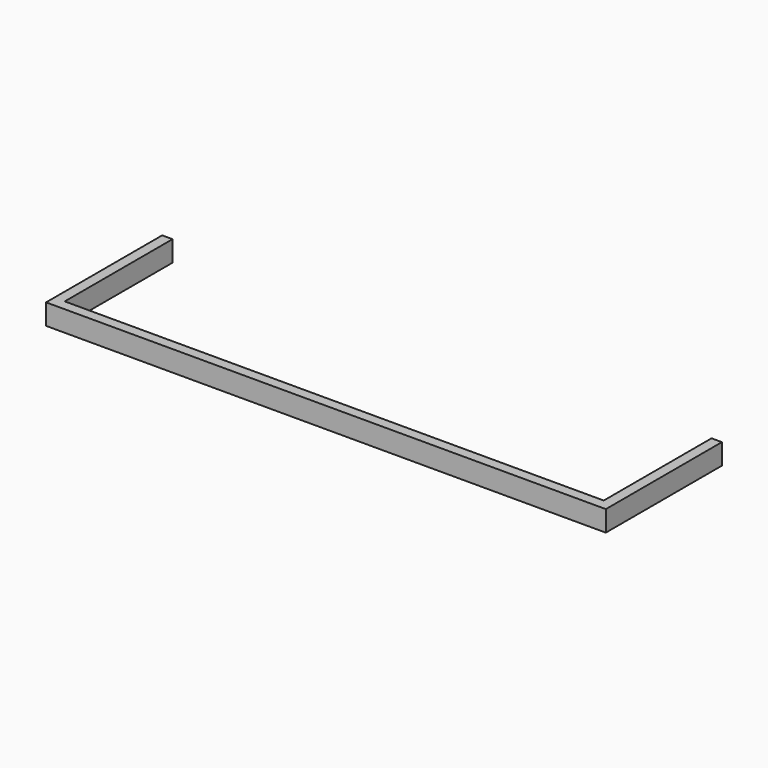
from build123d import *

# Parameters (mm, degrees)
F0_W          = 108
F0_H          = 30
F1_DEPTH      = 2
F3_DEPTH      = 39
F5_DEPTH      = 30.001
F6_DEPTH      = 4
F7_ANGLE      = -90
F8_T1_DEPTH   = 104
F8_T3_DEPTH   = 39
F8_T9_DEPTH   = 116.5
F8_T13_DEPTH  = 51.5
F8_T20_DEPTH  = 116.5
F8_T24_DEPTH  = 51.5
F9_R          = 2.55
F10_DEPTH     = 2.0010001
F15_TEXT_SIZE = 6.25
F16_DEPTH     = 0.7
F18_DEPTH     = 2


# Not quite as in the source:
# - a fillet or chamfer that OpenCascade refuses, or shapes differently, is made with other operations: its cross-section is extruded or revolved along the edge and cut away or added
# - a feature of the source that left no trace in its solid (it failed there, or was rolled back) is left out
# - Text() gives the source's letters only with a copy of the font that has no kerning and outlines rounded to 1/6400 em; it was checked with that copy


with BuildPart() as f1:
    # F0 (on Top) → F1 (new body)
    with BuildSketch(Plane.XY):
        with Locations((54, -15)):
            Rectangle(F0_W, F0_H)
    extrude(amount=-F1_DEPTH)

    # F2 (on face) → F3 (join)
    with BuildSketch(Plane(origin=(0, 0, -2), x_dir=(1, 0, 0), z_dir=(0, 0, -1))):
        Polygon((2, 28), (106, 28), (106, 2), (108, 2), (108, 30), (0, 30), (0, 2), (2, 2), align=None)
    extrude(amount=F3_DEPTH)

    # F4 (on face) → F5 (cut, through all)
    with BuildSketch(Plane.XZ.offset(30)):
        with BuildLine():
            Line((21.7352903846, -5.3176150288), (31.189246754, -24.36107081))
            ThreePointArc((31.189246754, -24.36107081), (22.5427599741, -36.7534160144), (37.0153844173, -32.408868279))
            Line((37.0153844173, -32.408868279), (35.7390828431, -20.9399661981))
            add(Edge.make_bspline(
                [(35.7390828431, -20.9399661981), (40.0774041837, -22.3301620555), (41.4828972701, -14.9319285827), (53.2948829776, -15.8111795219), (53.9903119206, -20.9399661981)],
                knots=[0, 0, 0, 0, 0.4737528897, 1, 1, 1, 1], degree=3))
            add(Edge.make_bspline(
                [(35.3899858892, -8.0947782844), (38.894245401, -7.2189187631), (48.5971156185, -8.2695706), (55.5558682276, -17.4074323859), (53.9903119206, -20.9399661981)],
                knots=[0, 0, 0, 0, 0.5069746376, 1, 1, 1, 1], degree=3))
            add(Edge.make_bspline(
                [(21.7352903846, -5.3176150288), (23.8003305692, -7.4651161077), (28.3369070804, -10.5817247057), (34.3228683985, -8.1395113196), (35.3899858892, -8.0947782844)],
                knots=[0, 0, 0, 0, 0.5306283003, 1, 1, 1, 1], degree=3))
        make_face()
    extrude(amount=-F5_DEPTH, mode=Mode.SUBTRACT)


with BuildPart() as f6:
    # F6 (new): a face of the model
    f6_faces = [f1.part.faces().sort_by_distance(p)[0] for p in [
        (54, -29.1157060545, -41),
    ]]
    extrude(f6_faces, amount=F6_DEPTH)


with BuildPart() as f1_1:
    # F7: moved
    add(f1.part.rotate(Axis((54, -30, -41), (-1, 0, 0)), F7_ANGLE))

    # F8: fillet of radius 5 on 3 edges, made by hand

    # F8_s2 → F8_t1 (join)
    with BuildSketch(Plane.YZ.offset(2)):
        with BuildLine():
            ThreePointArc((-69, -34), (-67.5355339059, -37.5355339059), (-64, -39))
            Line((-64, -39), (-64, -39.1))
            Line((-64, -39.1), (-69.1, -39.1))
            Line((-69.1, -39.1), (-69.1, -34))
            Line((-69.1, -34), (-69, -34))
        make_face()
    extrude(amount=F8_T1_DEPTH)

    # F8_s4 → F8_t3 (join)
    with BuildSketch(Plane.XZ.offset(30)):
        with BuildLine():
            ThreePointArc((7, -39), (3.4644660941, -37.5355339059), (2, -34))
            Line((2, -34), (1.9, -34))
            Line((1.9, -34), (1.9, -39.1))
            Line((1.9, -39.1), (7, -39.1))
            Line((7, -39.1), (7, -39))
        make_face()
        with BuildLine():
            ThreePointArc((101, -39), (104.5355339059, -37.5355339059), (106, -34))
            Line((106, -34), (106.1, -34))
            Line((106.1, -34), (106.1, -39.1))
            Line((106.1, -39.1), (101, -39.1))
            Line((101, -39.1), (101, -39))
        make_face()
    extrude(amount=F8_T3_DEPTH)


with BuildPart() as f8_tool7:
    # F8_s8 → F8_t9 (new body)
    with BuildSketch(Plane.YZ.offset(-10.5)):
        with BuildLine():
            ThreePointArc((-69, -34), (-67.5355339059, -37.5355339059), (-64, -39))
            Line((-64, -39), (-64, -39.1))
            Line((-64, -39.1), (-69.1, -39.1))
            Line((-69.1, -39.1), (-69.1, -34))
            Line((-69.1, -34), (-69, -34))
        make_face()
    extrude(amount=F8_T9_DEPTH)

    split(bisect_by=Plane.YZ.offset(2), keep=Keep.BOTTOM)


with BuildPart() as f8_tool11:
    # F8_s12 → F8_t13 (new body)
    with BuildSketch(Plane.XZ.offset(81.5)):
        with BuildLine():
            ThreePointArc((7, -39), (3.4644660941, -37.5355339059), (2, -34))
            Line((2, -34), (1.9, -34))
            Line((1.9, -34), (1.9, -39.1))
            Line((1.9, -39.1), (7, -39.1))
            Line((7, -39.1), (7, -39))
        make_face()
    extrude(amount=-F8_T13_DEPTH)

    split(bisect_by=Plane.XZ.offset(69), keep=Keep.TOP)


with BuildPart() as f8_tool7_1:
    add(f8_tool7.part)

    # F8_t15: intersect F8_tool11
    add(f8_tool11.part, mode=Mode.INTERSECT)


with BuildPart() as f1_2:
    add(f1_1.part)

    # F8_t5: union F8_tool7
    add(f8_tool7_1.part)


with BuildPart() as f8_tool18:
    # F8_s19 → F8_t20 (new body)
    with BuildSketch(Plane.YZ.offset(2)):
        with BuildLine():
            ThreePointArc((-69, -34), (-67.5355339059, -37.5355339059), (-64, -39))
            Line((-64, -39), (-64, -39.1))
            Line((-64, -39.1), (-69.1, -39.1))
            Line((-69.1, -39.1), (-69.1, -34))
            Line((-69.1, -34), (-69, -34))
        make_face()
    extrude(amount=F8_T20_DEPTH)

    split(bisect_by=Plane.YZ.offset(106), keep=Keep.TOP)


with BuildPart() as f8_tool22:
    # F8_s23 → F8_t24 (new body)
    with BuildSketch(Plane.XZ.offset(81.5)):
        with BuildLine():
            ThreePointArc((101, -39), (104.5355339059, -37.5355339059), (106, -34))
            Line((106, -34), (106.1, -34))
            Line((106.1, -34), (106.1, -39.1))
            Line((106.1, -39.1), (101, -39.1))
            Line((101, -39.1), (101, -39))
        make_face()
    extrude(amount=-F8_T24_DEPTH)

    split(bisect_by=Plane.XZ.offset(69), keep=Keep.TOP)


with BuildPart() as f8_tool18_1:
    add(f8_tool18.part)

    # F8_t26: intersect F8_tool22
    add(f8_tool22.part, mode=Mode.INTERSECT)


with BuildPart() as f1_3:
    add(f1_2.part)

    # F8_t16: union F8_tool18
    add(f8_tool18_1.part)

    # F9 (on face) → F10 (cut, through all)
    with BuildSketch(Plane(origin=(0, -69, 0), x_dir=(-1, 0, 0), z_dir=(0, 1, 0))):
        with BuildLine():
            Line((-48, -29.9), (-46, -29.9))
            ThreePointArc((-46, -29.9), (-44.5857864376, -29.3142135624), (-44, -27.9))
            Line((-44, -27.9), (-44, -27.8))
            ThreePointArc((-44, -27.8), (-44.5857864376, -26.3857864376), (-46, -25.8))
            Line((-46, -25.8), (-50, -25.8))
            ThreePointArc((-50, -25.8), (-51.4142135624, -26.3857864376), (-52, -27.8))
            Line((-52, -27.8), (-52, -27.9))
            ThreePointArc((-52, -27.9), (-51.4142135624, -29.3142135624), (-50, -29.9))
            Line((-50, -29.9), (-48, -29.9))
        make_face()
        with Locations((-22.5, -27.4)):
            Circle(F9_R)
    extrude(amount=-F10_DEPTH, mode=Mode.SUBTRACT)

    # F15 (on face) → F16 (cut)
    with BuildSketch(Plane.XZ.offset(71)):
        with Locations((15.8969726562, -37)):
            Text('AUX', F15_TEXT_SIZE, font='Open Sans', font_style=FontStyle.BOLD, text_align=(TextAlign.LEFT, TextAlign.BOTTOM))
        with Locations((36.0439453125, -37)):
            Text('OFF/ON', F15_TEXT_SIZE, font='Open Sans', font_style=FontStyle.BOLD, text_align=(TextAlign.LEFT, TextAlign.BOTTOM))
    extrude(amount=-F16_DEPTH, mode=Mode.SUBTRACT)

    # F17 (on face) → F18 (cut, through all)
    with BuildSketch(Plane.YZ.offset(108)):
        with BuildLine():
            Line((-32.9, -15.3), (-32.9, -13))
            Line((-32.9, -13), (-37.1, -13))
            Line((-37.1, -13), (-37.1, -15.3))
            ThreePointArc((-37.1, -15.3), (-36.5142135624, -16.7142135624), (-35.1, -17.3))
            Line((-35.1, -17.3), (-34.9, -17.3))
            ThreePointArc((-34.9, -17.3), (-33.4857864376, -16.7142135624), (-32.9, -15.3))
        make_face()
    extrude(amount=-F18_DEPTH, mode=Mode.SUBTRACT)


with BuildPart() as f19_1:
    # F19: copy of F6
    add(f6.part.moved(Location((0, 46.18289, 0))))


solid = f6.part
